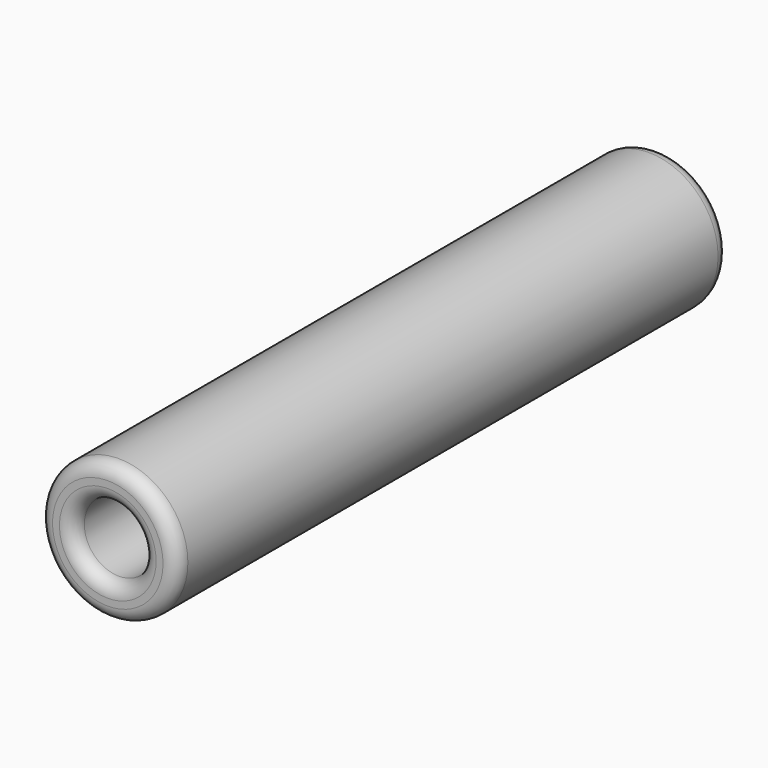
from build123d import *

# Parameters (mm, degrees)
F0_R     = 12.7
F1_DEPTH = 63.5
F3_D     = 12.7
F4_R     = 2.54


with BuildPart() as f1:
    # F0 (on Front) → F1 (new body, symmetric)
    with BuildSketch(Plane.XZ):
        Circle(F0_R)
    extrude(amount=F1_DEPTH, both=True)

    # F3 (through all)
    with Locations(Plane(origin=(0, 63.5, 0), x_dir=(-1, 0, 0), z_dir=(0, 1, 0))):
        with Locations((0, 0)):
            Hole(F3_D / 2)

    # F4
    f4_edges = [f1.edges().sort_by_distance(p)[0] for p in [
        (-12.7, -63.5, 0),
        (-12.7, 63.5, 0),
        (6.35, 63.5, 0),
        (6.35, -63.5, 0),
    ]]
    fillet(f4_edges, radius=F4_R)


solid = f1.part
